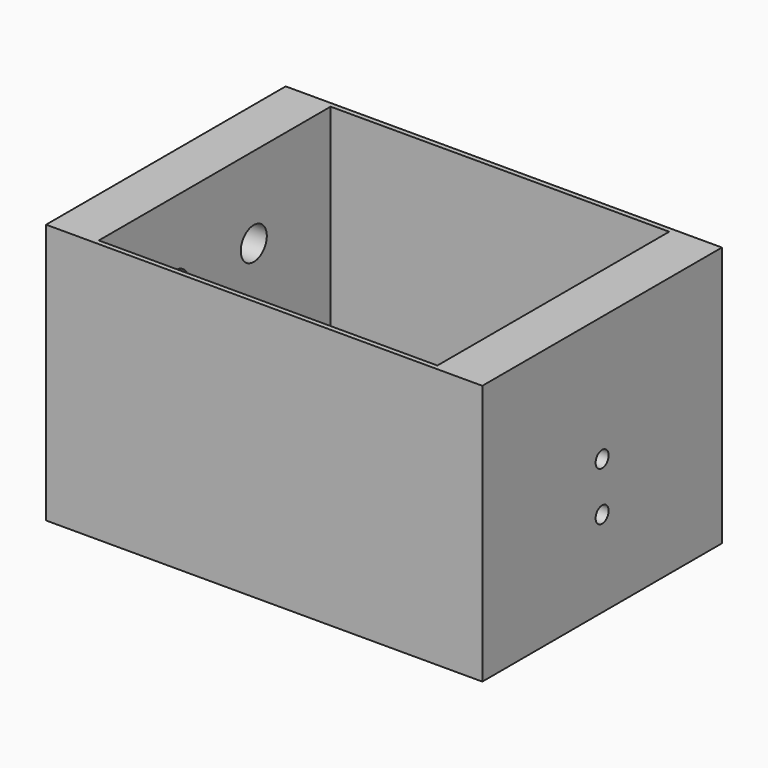
from build123d import *

# Parameters (mm, degrees)
F0_R      = 25.5
F1_DEPTH  = 2
F0_R_2    = 5
F2_DEPTH  = 5
F3_DEPTH  = 160
F4_DEPTH  = 40
F5_R      = 5
F6_DEPTH  = 30.3
F7_DEPTH  = 30
F8_DEPTH  = 10
F9_R      = 10
F10_DEPTH = 30


# Not quite as in the source:
# - a feature names something its author has since deleted; it is built from what else it names


with BuildPart() as f1:
    # F0 (on Top) → F1 (new body)
    with BuildSketch(Plane.XY):
        Circle(F0_R)
    extrude(amount=F1_DEPTH)

    # F0 (on Top) → F8 (cut)
    with BuildSketch(Plane.XY):
        with BuildLine():
            Line((94, -10), (94, 0))
            Line((94, 0), (94, 10))
            ThreePointArc((94, 10), (90, 14), (86, 10))
            Line((86, 10), (86, -10))
            ThreePointArc((86, -10), (90, -14), (94, -10))
        make_face()
    extrude(amount=F8_DEPTH, mode=Mode.SUBTRACT)


with BuildPart() as f2:
    # F0 (on Top) → F2 (new body)
    with BuildSketch(Plane.XY):
        Polygon((100, -85), (100, 0), (100, 85), (-100, 85), (-100, -85), align=None)
        with Locations((-94, 0)):
            Circle(F0_R_2, mode=Mode.SUBTRACT)
        Circle(F0_R, mode=Mode.SUBTRACT)
        with BuildLine():
            Line((94, 10), (94, 0))
            Line((94, 0), (94, -10))
            ThreePointArc((94, -10), (90, -14), (86, -10))
            Line((86, -10), (86, 10))
            ThreePointArc((86, 10), (90, 14), (94, 10))
        make_face(mode=Mode.SUBTRACT)
    extrude(amount=F2_DEPTH)


with BuildPart() as f3:
    # F0 (on Top) → F3 (new body)
    with BuildSketch(Plane.XY):
        Polygon((-134, -92), (134, -92), (134, 0), (134, 92), (-134, 92), align=None)
        Polygon((104, 89), (104, 0), (104, -89), (-104, -89), (-104, 89), align=None, mode=Mode.SUBTRACT)
    extrude(amount=F3_DEPTH)

    # F5 (on face) → F6 (cut)
    with BuildSketch(Plane.YZ.offset(134)):
        with Locations((0, 83)):
            Circle(F5_R)
    extrude(amount=-F6_DEPTH, mode=Mode.SUBTRACT)

    # F5 (on face) → F7 (cut)
    with BuildSketch(Plane.YZ.offset(134)):
        with Locations((0, 53)):
            Circle(F5_R)
    extrude(amount=-F7_DEPTH, mode=Mode.SUBTRACT)

    # F9 (on face) → F10 (cut, through all)
    with BuildSketch(Plane(origin=(-134, 0, 0), x_dir=(0, -1, 0), z_dir=(-1, 0, 0))):
        with Locations((-30, 110)):
            Circle(F9_R)
        with Locations((30, 110)):
            Circle(F9_R)
        with Locations((-30, 50)):
            Circle(F9_R)
        with Locations((30, 50)):
            Circle(F9_R)
    extrude(amount=-F10_DEPTH, mode=Mode.SUBTRACT)


with BuildPart() as f4:
    # F0 (on Top) → F4 (new body)
    with BuildSketch(Plane.XY):
        Polygon((104, -89), (104, 0), (104, 89), (-104, 89), (-104, -89), align=None)
        Polygon((100, 85), (100, 0), (100, -85), (-100, -85), (-100, 85), align=None, mode=Mode.SUBTRACT)
    extrude(amount=F4_DEPTH)


solid = Compound([f1.part, f2.part, f3.part, f4.part])
